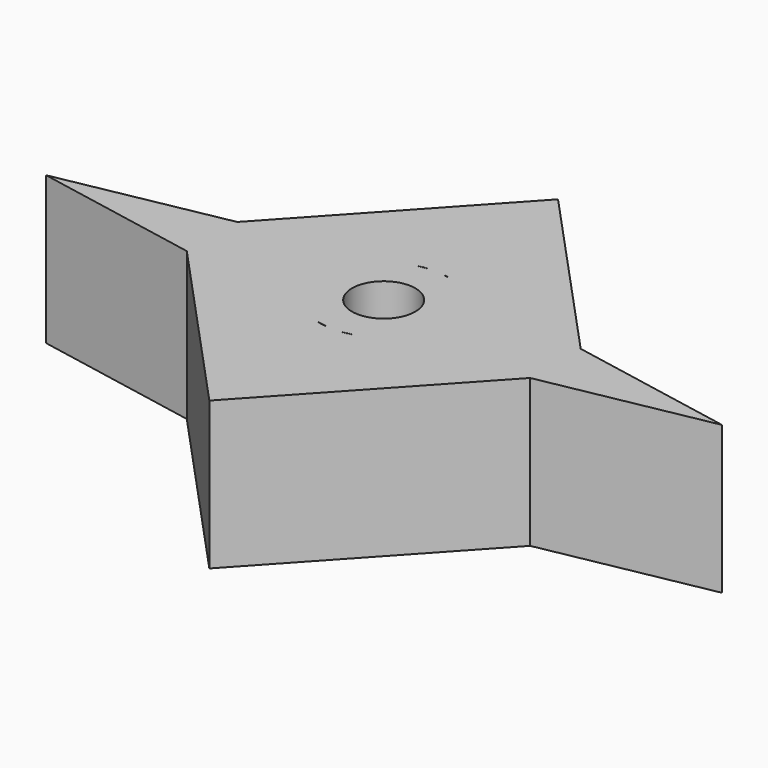
from build123d import *

# Parameters (mm, degrees)
F0_R     = 9.525
F1_DEPTH = 44.45
F2_DEPTH = 44.45
F3_DEPTH = 44.45
F4_DEPTH = 44.45
F5_DEPTH = 44.45
F6_DEPTH = 44.45
F7_DEPTH = 44.45
F8_DEPTH = 25.4
F9_DEPTH = 19.05


with BuildPart() as f1:
    # F0 (on Top) → F1 (new body)
    with BuildSketch(Plane.XY):
        with BuildLine():
            Line((5.1747410867, 18.3336999726), (1.9060083062, 18.9544093112))
            ThreePointArc((1.9060083062, 18.9544093112), (0.0969078237, 19.0497535122), (-1.7130690518, 18.9728198859))
            Line((-1.7130690518, 18.9728198859), (-5.3677419125, 18.2781248152))
            ThreePointArc((-5.3677419125, 18.2781248152), (-19.05, 0), (-5.3677419125, -18.2781248152))
            Line((-5.3677419125, -18.2781248152), (-1.7130690518, -18.9728198859))
            ThreePointArc((-1.7130690518, -18.9728198859), (0.0969078237, -19.0497535122), (1.9060083062, -18.9544093112))
            Line((1.9060083062, -18.9544093112), (5.1747410867, -18.3336999726))
            ThreePointArc((5.1747410867, -18.3336999726), (15.1901500602, -11.4961663675), (19.05, 0))
            ThreePointArc((19.05, 0), (15.1901500602, 11.4961663675), (5.1747410867, 18.3336999726))
        make_face()
        Circle(F0_R, mode=Mode.SUBTRACT)
        with BuildLine():
            Line((51.6444474156, 9.5094299521), (5.1747410867, 18.3336999726))
            ThreePointArc((5.1747410867, 18.3336999726), (15.1901500602, 11.4961663675), (19.05, 0))
            ThreePointArc((19.05, 0), (15.1901500602, -11.4961663675), (5.1747410867, -18.3336999726))
            Line((5.1747410867, -18.3336999726), (51.6444474156, -9.5094299521))
            Line((51.6444474156, -9.5094299521), (101.722291385, 0))
            Line((101.722291385, 0), (51.6444474156, 9.5094299521))
        make_face()
    extrude(amount=F1_DEPTH)

    # F0 (on Top) → F2 (join)
    with BuildSketch(Plane.XY):
        with BuildLine():
            Line((0, 65.538806632), (1.9060083062, 18.9544093112))
            ThreePointArc((1.9060083062, 18.9544093112), (3.5539517459, 18.7155530773), (5.1747410867, 18.3336999726))
            Line((5.1747410867, 18.3336999726), (51.6444474156, 9.5094299521))
            Line((51.6444474156, 9.5094299521), (0, 65.538806632))
        make_face()
    extrude(amount=F2_DEPTH)

    # F0 (on Top) → F3 (join)
    with BuildSketch(Plane.XY):
        with BuildLine():
            ThreePointArc((-5.3677419125, -18.2781248152), (-19.05, 0), (-5.3677419125, 18.2781248152))
            Line((-5.3677419125, 18.2781248152), (-51.6194616924, 9.486409943))
            Line((-51.6194616924, 9.486409943), (-101.5258543329, 0))
            Line((-101.5258543329, 0), (-51.6194616924, -9.486409943))
            Line((-51.6194616924, -9.486409943), (-5.3677419125, -18.2781248152))
        make_face()
    extrude(amount=F3_DEPTH)

    # F0 (on Top) → F4 (join)
    with BuildSketch(Plane.XY):
        with BuildLine():
            ThreePointArc((1.9060083062, -18.9544093112), (0.0969078237, -19.0497535122), (-1.7130690518, -18.9728198859))
            Line((-1.7130690518, -18.9728198859), (0, -65.538806632))
            Line((0, -65.538806632), (1.9060083062, -18.9544093112))
        make_face()
    extrude(amount=F4_DEPTH)

    # F0 (on Top) → F5 (join)
    with BuildSketch(Plane.XY):
        with BuildLine():
            ThreePointArc((-1.7130690518, 18.9728198859), (0.0969078237, 19.0497535122), (1.9060083062, 18.9544093112))
            Line((1.9060083062, 18.9544093112), (0, 65.538806632))
            Line((0, 65.538806632), (-1.7130690518, 18.9728198859))
        make_face()
    extrude(amount=F5_DEPTH)

    # F0 (on Top) → F6 (join)
    with BuildSketch(Plane.XY):
        with BuildLine():
            ThreePointArc((-1.7130690518, -18.9728198859), (-3.5574037286, -18.7148972402), (-5.3677419125, -18.2781248152))
            Line((-5.3677419125, -18.2781248152), (-51.6194616924, -9.486409943))
            Line((-51.6194616924, -9.486409943), (0, -65.538806632))
            Line((0, -65.538806632), (-1.7130690518, -18.9728198859))
        make_face()
        with BuildLine():
            Line((51.6444474156, -9.5094299521), (5.1747410867, -18.3336999726))
            ThreePointArc((5.1747410867, -18.3336999726), (3.5539517459, -18.7155530773), (1.9060083062, -18.9544093112))
            Line((1.9060083062, -18.9544093112), (0, -65.538806632))
            Line((0, -65.538806632), (51.6444474156, -9.5094299521))
        make_face()
    extrude(amount=F6_DEPTH)

    # F0 (on Top) → F7 (join)
    with BuildSketch(Plane.XY):
        with BuildLine():
            Line((0, 65.538806632), (1.9060083062, 18.9544093112))
            ThreePointArc((1.9060083062, 18.9544093112), (3.5539517459, 18.7155530773), (5.1747410867, 18.3336999726))
            Line((5.1747410867, 18.3336999726), (51.6444474156, 9.5094299521))
            Line((51.6444474156, 9.5094299521), (0, 65.538806632))
        make_face()
    extrude(amount=F7_DEPTH)

    # F0 (on Top) → F8 (join)
    with BuildSketch(Plane.XY):
        with BuildLine():
            ThreePointArc((-5.3677419125, 18.2781248152), (-3.5574037286, 18.7148972402), (-1.7130690518, 18.9728198859))
            Line((-1.7130690518, 18.9728198859), (0, 65.538806632))
            Line((0, 65.538806632), (-51.6194616924, 9.486409943))
            Line((-51.6194616924, 9.486409943), (-5.3677419125, 18.2781248152))
        make_face()
    extrude(amount=F8_DEPTH)

    # F9 (add): a face of the model
    f9_faces = [f1.faces().sort_by_distance(p)[0] for p in [
        (-17.7802963079, 31.335159678, 25.4),
    ]]
    extrude(f9_faces, amount=F9_DEPTH)


solid = f1.part
